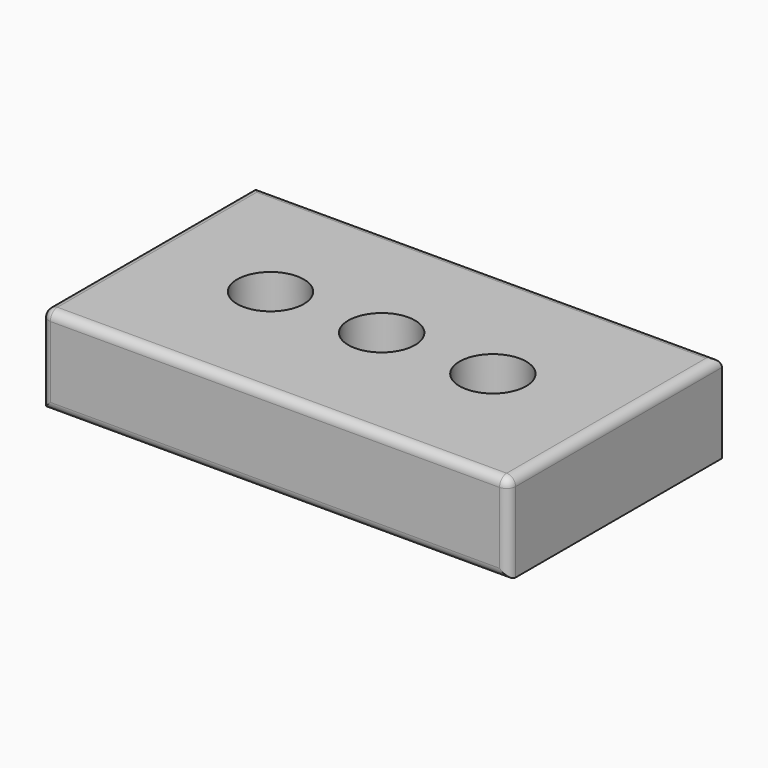
from build123d import *

# Parameters (mm, degrees)
F0_W     = 266.7
F0_H     = 152.4
F0_R     = 19.05
F1_DEPTH = 50.8
F2_R     = 5.08


# Not quite as in the source:
# - a feature names something its author has since deleted; it is built from what else it names


with BuildPart() as f1:
    # F0 (on Top) → F1 (new body)
    with BuildSketch(Plane.XY):
        Rectangle(F0_W, F0_H)
        with Locations((-63.5, 0)):
            Circle(F0_R, mode=Mode.SUBTRACT)
        Circle(F0_R, mode=Mode.SUBTRACT)
        with Locations((63.5, 0)):
            Circle(F0_R, mode=Mode.SUBTRACT)
    extrude(amount=-F1_DEPTH)

    # F2
    f2_edges = [f1.edges().sort_by_distance(p)[0] for p in [
        (-133.35, 0, 0),
        (0, 76.2, 0),
        (133.35, 0, 0),
        (-133.35, -76.2, -25.4),
        (133.35, -76.2, -25.4),
        (0, -76.2, 0),
        (0, -76.2, -50.8),
    ]]
    fillet(f2_edges, radius=F2_R)


solid = f1.part
